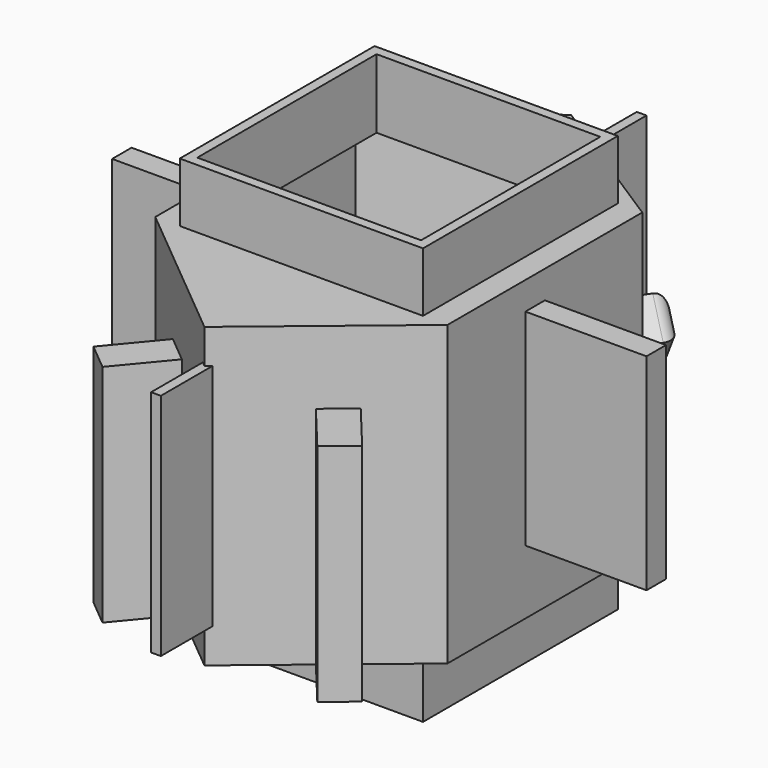
from build123d import *

# Parameters (mm, degrees)
F0_W         = 6.3855407542
F0_H         = 63.4993868415
F3_DEPTH     = 38.862
F0_W_2       = 63.4289184916
F4_DEPTH     = 54.356
F5_DEPTH     = 1.27
F1_W         = 40.2324178779
F1_H         = 53.7178423256
F6_DEPTH     = 6.35
F7_T         = 2.54
F7_T3_DEPTH  = 68.5793868415
F7_T5_DEPTH  = 68.5089184916
F7_T7_DEPTH  = 6.5892994553
F7_T9_DEPTH  = 64.8371359067
F7_T11_DEPTH = 6.5892994553
F7_T13_DEPTH = 58.7978423256
F7_T15_DEPTH = 11.43
F7_T17_DEPTH = 6.7300617299
F7_T19_DEPTH = 6.7300617299
F7_T21_DEPTH = 6.7300617299
F7_T23_DEPTH = 6.7300617299
F7_T25_DEPTH = 6.5892994553
F7_T27_DEPTH = 6.5892994553
F9_DEPTH     = 5.334
F11_DEPTH    = 13.208
F12_R        = 3.6792614691
F13_W        = 9.1328918934
F13_H        = 58.7153472006
F14_DEPTH    = 16.51


# Not quite as in the source:
# - a pattern or mirror of a feature is missing from the dataset's text; its kind, count and spacing are read off the source's solid
# - a shell that OpenCascade refuses in one call is made with other operations: the cavity is built on its own and cut out


with BuildPart() as f3:
    # F0 (on Top) → F3 (new body, symmetric)
    with BuildSketch(Plane.XY):
        Polygon((31.7144592458, 31.7496934207), (38.1, 31.7496934207), (0, 56.2155136837), (-38.1, 31.7496934207), (-31.7144592458, 31.7496934207), align=None)
        Polygon((0, -63.3538599396), (38.1, -31.7496934207), (31.7144592458, -31.7496934207), (-31.7144592458, -31.7496934207), (-38.1, -31.7496934207), align=None)
        with Locations((-34.9072296229, 0)):
            Rectangle(F0_W, F0_H)
        with Locations((34.9072296229, 0)):
            Rectangle(F0_W, F0_H)
    extrude(amount=F3_DEPTH, both=True)

    # F0 (on Top) → F4 (join, symmetric)
    with BuildSketch(Plane.XY):
        Rectangle(F0_W_2, F0_H)
    extrude(amount=F4_DEPTH, both=True)

    # F2 (on Right) → F5 (join, symmetric)
    with BuildSketch(Plane.YZ):
        Polygon((52.2253494244, 29.8785679533), (52.2253494244, 0), (52.2253494244, -29.8785679533), (79.1521295905, -29.8785679533), (79.1521295905, 29.8785679533), align=None)
        Polygon((-52.2253494244, -29.8785679533), (-52.2253494244, 0), (-52.2253494244, 29.8785679533), (-79.1521295905, 29.8785679533), (-79.1521295905, -29.8785679533), align=None)
    extrude(amount=F5_DEPTH, both=True)

    # F1 (on Front) → F6 (join)
    with BuildSketch(Plane.XZ):
        with Locations((49.563405104, 4.7380579636)):
            Rectangle(F1_W, F1_H)
        with Locations((-49.563405104, 4.7380579636)):
            Rectangle(F1_W, F1_H)
    extrude(amount=F6_DEPTH)

    # F7: shell of thickness 2.54, made by hand


with BuildPart() as f7_core1:
    # F7_t2: copy of F3
    add(f3.part)

    # the walls: a layer under each face that stays
    f7_faces = [f7_core1.faces().sort_by_distance(p)[0] for p in [
        (-31.7144592458, 0, -46.609),
        (0, 31.7496934207, -46.609),
        (-25.4, 36.2872847465, -38.862),
        (0, -31.7496934207, -46.609),
        (0, 0, -54.356),
        (31.7144592458, 0, -46.609),
        (-19.05, 43.9826035522, 0),
        (-38.1, 21.1664622805, -25.908),
        (-19.05, -47.5517766802, 0),
        (19.05, -47.5517766802, 0),
        (38.1, -21.1664622805, -25.908),
        (19.05, 43.9826035522, 0),
        (0, 67.276057966, -29.8785679533),
        (-1.27, 67.276057966, 0),
        (0, 67.276057966, 29.8785679533),
        (-25.4, 36.2872847465, 38.862),
        (-53.8898070215, 0, 4.7380579636),
        (-53.8898070215, -3.175, -22.1208631992),
        (-53.8898070215, -6.35, 4.7380579636),
        (-53.8898070215, -3.175, 31.5969791263),
        (0, -70.7262586564, 29.8785679533),
        (-1.27, -70.7262586564, 0),
        (0, -70.7262586564, -29.8785679533),
        (1.27, -70.7262586564, 0),
        (53.8898070215, 0, 4.7380579636),
        (53.8898070215, -3.175, 31.5969791263),
        (53.8898070215, -6.35, 4.7380579636),
        (53.8898070215, -3.175, -22.1208631992),
        (1.27, 67.276057966, 0),
        (0, 79.1521295905, 0),
        (0, -31.7496934207, 46.609),
        (-31.7144592458, 0, 46.609),
        (0, 31.7496934207, 46.609),
        (31.7144592458, 0, 46.609),
        (-69.679614043, -3.175, 4.7380579636),
        (0, -79.1521295905, 0),
        (69.679614043, -3.175, 4.7380579636),
    ]]
    thicken(f7_faces, amount=-F7_T, mode=Mode.SUBTRACT)

    # F7_s4 → F7_t3 (cut)
    with BuildSketch(Plane.XZ.offset(-34.2896934207)):
        Polygon((-31.7398592458, -38.8874), (-29.1744592458, -38.862), (-29.1744592458, -36.322), (-31.7144592458, -36.322), align=None)
        Polygon((31.7398592458, -38.8874), (31.7144592458, -36.322), (29.1744592458, -36.322), (29.1744592458, -38.862), align=None)
        Polygon((-31.7398592458, 38.8874), (-31.7144592458, 36.322), (-29.1744592458, 36.322), (-29.1744592458, 38.862), align=None)
        Polygon((31.7398592458, 38.8874), (31.7144592458, 36.322), (29.1744592458, 36.322), (29.1744592458, 38.862), align=None)
    extrude(amount=F7_T3_DEPTH, mode=Mode.SUBTRACT)

    # F7_s6 → F7_t5 (cut)
    with BuildSketch(Plane.YZ.offset(-34.2544592458)):
        Polygon((31.7750934207, -38.8874), (29.2096934207, -38.862), (29.2096934207, -36.322), (31.7496934207, -36.322), align=None)
        Polygon((-31.7750934207, -38.8874), (-31.7496934207, -36.322), (-29.2096934207, -36.322), (-29.2096934207, -38.862), align=None)
        Polygon((-31.7750934207, 38.8874), (-31.7496934207, 36.322), (-29.2096934207, 36.322), (-29.2096934207, 38.862), align=None)
        Polygon((31.7750934207, 38.8874), (31.7496934207, 36.322), (29.2096934207, 36.322), (29.2096934207, 38.862), align=None)
    extrude(amount=F7_T5_DEPTH, mode=Mode.SUBTRACT)

    # F7_s8 → F7_t7 (cut)
    with BuildSketch(Plane(origin=(27.6965031812, 17.7852406494, 0), x_dir=(0, 0, 1), z_dir=(-0.8414499823, -0.5403350139, 0))):
        Polygon((-29.9039679533, 47.3279429967), (-29.8785679533, 44.7625429967), (-27.3385679533, 44.7625429967), (-27.3385679533, 47.3025429967), align=None)
    extrude(amount=F7_T7_DEPTH, mode=Mode.SUBTRACT)

    # F7_s10 → F7_t9 (cut)
    with BuildSketch(Plane.XY.offset(-32.4185679533)):
        Polygon((-1.3091245094, 55.4213591711), (0.1024509352, 53.2627033864), (1.27, 54.0124421152), (1.27, 55.3999863416), align=None)
        Polygon((-1.3116164808, -62.319937294), (0.3516480774, -60.3454305583), (1.27, -61.1072086971), (1.27, -62.3003877224), align=None)
        Polygon((1.3116164808, -62.319937294), (-0.3516480774, -60.3454305583), (-1.27, -61.1072086971), (-1.27, -62.3003877224), align=None)
        Polygon((1.3091245094, 55.4213591711), (-0.1024509352, 53.2627033864), (-1.27, 54.0124421152), (-1.27, 55.3999863416), align=None)
    extrude(amount=F7_T9_DEPTH, mode=Mode.SUBTRACT)

    # F7_s12 → F7_t11 (cut)
    with BuildSketch(Plane(origin=(22.1519372709, 14.2248114369, 0), x_dir=(0, 0, 1), z_dir=(0.8414499823, 0.5403350139, 0))):
        Polygon((29.9039679533, -47.3279429967), (29.8785679533, -44.7625429967), (27.3385679533, -44.7625429967), (27.3385679533, -47.3025429967), align=None)
    extrude(amount=F7_T11_DEPTH, mode=Mode.SUBTRACT)

    # F7_s14 → F7_t13 (cut)
    with BuildSketch(Plane.XY.offset(-24.6608631992)):
        Polygon((-38.1254, 0.0254), (-35.56, 0), (-35.56, -2.54), (-38.1, -2.54), align=None)
        Polygon((-38.1254, -6.3754), (-35.56, -6.35), (-35.56, -3.81), (-38.1, -3.81), align=None)
        Polygon((38.1254, 0.0254), (35.56, 0), (35.56, -2.54), (38.1, -2.54), align=None)
        Polygon((38.1254, -6.3754), (35.56, -6.35), (35.56, -3.81), (38.1, -3.81), align=None)
    extrude(amount=F7_T13_DEPTH, mode=Mode.SUBTRACT)

    # F7_s16 → F7_t15 (cut)
    with BuildSketch(Plane.XZ.offset(-2.54)):
        Polygon((-38.1254, -22.1462631992), (-35.56, -22.1208631992), (-35.56, -19.5808631992), (-38.1, -19.5808631992), align=None)
        Polygon((-38.1254, 31.6223791263), (-35.56, 31.5969791263), (-35.56, 29.0569791263), (-38.1, 29.0569791263), align=None)
        Polygon((38.1254, 31.6223791263), (35.56, 31.5969791263), (35.56, 29.0569791263), (38.1, 29.0569791263), align=None)
        Polygon((38.1254, -22.1462631992), (35.56, -22.1208631992), (35.56, -19.5808631992), (38.1, -19.5808631992), align=None)
    extrude(amount=F7_T15_DEPTH, mode=Mode.SUBTRACT)

    # F7_s18 → F7_t17 (cut)
    with BuildSketch(Plane(origin=(33.0864182791, -27.4453719897, 0), x_dir=(0, 0, 1), z_dir=(-0.7696681748, 0.638444125, 0))):
        Polygon((29.9039679533, -48.7868497466), (29.8785679533, -46.2214497466), (27.3385679533, -46.2214497466), (27.3385679533, -48.7614497466), align=None)
    extrude(amount=F7_T17_DEPTH, mode=Mode.SUBTRACT)

    # F7_s20 → F7_t19 (cut)
    with BuildSketch(Plane(origin=(27.9065039511, -23.1486036176, 0), x_dir=(0, 0, 1), z_dir=(0.7696681748, -0.638444125, 0))):
        Polygon((-29.9039679533, 48.7868497466), (-29.8785679533, 46.2214497466), (-27.3385679533, 46.2214497466), (-27.3385679533, 48.7614497466), align=None)
    extrude(amount=F7_T19_DEPTH, mode=Mode.SUBTRACT)

    # F7_s22 → F7_t21 (cut)
    with BuildSketch(Plane(origin=(-33.0864182791, -27.4453719897, 0), x_dir=(0, 0, 1), z_dir=(0.7696681748, 0.638444125, 0))):
        Polygon((-29.9039679533, 48.7868497466), (-29.8785679533, 46.2214497466), (-27.3385679533, 46.2214497466), (-27.3385679533, 48.7614497466), align=None)
    extrude(amount=F7_T21_DEPTH, mode=Mode.SUBTRACT)

    # F7_s24 → F7_t23 (cut)
    with BuildSketch(Plane(origin=(-27.9065039511, -23.1486036176, 0), x_dir=(0, 0, 1), z_dir=(-0.7696681748, -0.638444125, 0))):
        Polygon((29.9039679533, -48.7868497466), (29.8785679533, -46.2214497466), (27.3385679533, -46.2214497466), (27.3385679533, -48.7614497466), align=None)
    extrude(amount=F7_T23_DEPTH, mode=Mode.SUBTRACT)

    # F7_s26 → F7_t25 (cut)
    with BuildSketch(Plane(origin=(-27.6965031812, 17.7852406494, 0), x_dir=(0, 0, 1), z_dir=(0.8414499823, -0.5403350139, 0))):
        Polygon((29.9039679533, -47.3279429967), (29.8785679533, -44.7625429967), (27.3385679533, -44.7625429967), (27.3385679533, -47.3025429967), align=None)
    extrude(amount=F7_T25_DEPTH, mode=Mode.SUBTRACT)

    # F7_s28 → F7_t27 (cut)
    with BuildSketch(Plane(origin=(-22.1519372709, 14.2248114369, 0), x_dir=(0, 0, 1), z_dir=(-0.8414499823, 0.5403350139, 0))):
        Polygon((-29.9039679533, 47.3279429967), (-29.8785679533, 44.7625429967), (-27.3385679533, 44.7625429967), (-27.3385679533, 47.3025429967), align=None)
    extrude(amount=F7_T27_DEPTH, mode=Mode.SUBTRACT)


with BuildPart() as f3_1:
    add(f3.part)

    # what is left inside the walls is the cavity
    f7_cavity = [f7_core1.part.solids().sort_by_distance(p)[0] for p in [
        (-35.5346, -0.097183, -12.107333),
    ]]
    add(f7_cavity, mode=Mode.SUBTRACT)

    # F8 (on face) → F9 (join)
    with BuildSketch(Plane(origin=(0, 0, -54.356), x_dir=(1, 0, 0), z_dir=(0, 0, -1))):
        Polygon((23.1188687153, -13.7063056679), (0.3105745427, 26.8746804482), (-23.4294432581, -13.1683747803), align=None)
    extrude(amount=F9_DEPTH)

    # F10 (on face) → F11 (join)
    with BuildSketch(Plane(origin=(25.559220226, 39.8027239695, 0), x_dir=(-0.8414499823, 0.5403350139, 0), z_dir=(0.5403350139, 0.8414499823, 0))):
        Polygon((6.6651697271, -9.5054283738), (6.6651697271, 0), (6.6651697271, 8.0630239099), (0, 0), align=None)
        Polygon((6.6651697271, 8.0630239099), (6.6651697271, 0), (6.6651697271, -9.5054283738), (12.8076681867, 0), align=None)
    f11 = extrude(amount=F11_DEPTH)

    # F11_copies: F11 across plane
    add(f11.mirror(Plane(origin=(0, 0, 0), x_dir=(0, 0, -1), z_dir=(-1, 0, 0))))

    # F12
    f12_edges = [f3_1.edges().sort_by_distance(p)[0] for p in [
        (29.891762, 52.717308, 4.031512),
        (24.503256, 56.177523, -4.752714),
        (24.503256, 56.177523, 4.031512),
        (29.891762, 52.717308, -4.752714),
        (-24.503256, 56.177523, 4.031512),
        (-24.503256, 56.177523, -4.752714),
        (-29.891762, 52.717308, -4.752714),
        (-29.891762, 52.717308, 4.031512),
    ]]
    fillet(f12_edges, radius=F12_R)


with BuildPart() as f14:
    # F13 (on face) → F14 (new body)
    with BuildSketch(Plane(origin=(-31.1314611151, -37.5301360273, 0), x_dir=(0.7696681748, -0.638444125, 0), z_dir=(-0.638444125, -0.7696681748, 0))):
        with Locations((13.183509931, -9.5102321357)):
            Rectangle(F13_W, F13_H)
    extrude(amount=F14_DEPTH)


with BuildPart() as f15_1:
    # F15: instance of F14
    add(f14.part.mirror(Plane.YZ))


solid = Compound([f3_1.part, f14.part, f15_1.part])
